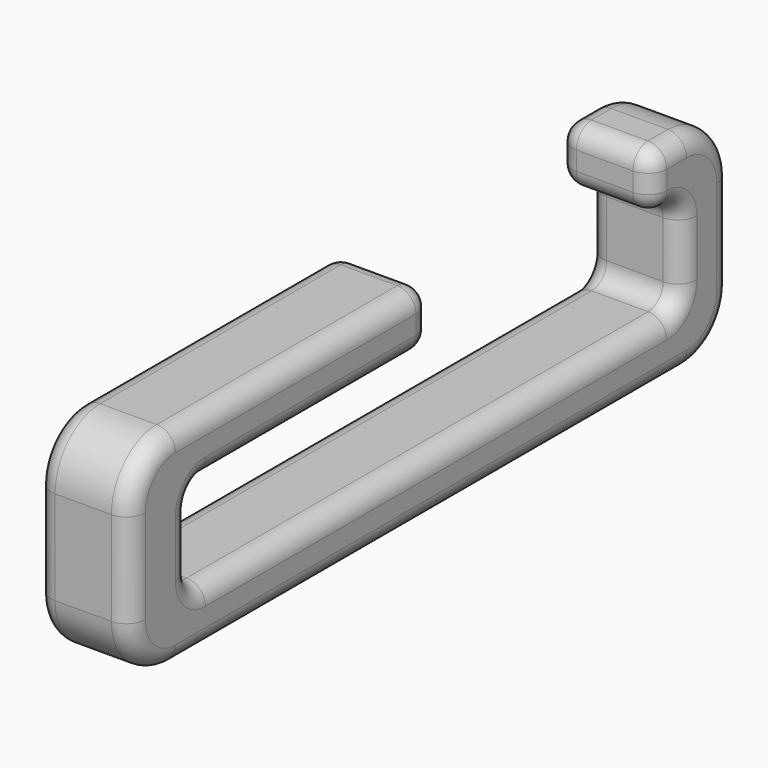
from build123d import *

# Parameters (mm, degrees)
F0_W     = 5
F0_H     = 3.3166247904
F0_H_2   = 16
F0_H_3   = 14.6833752096
F0_H_4   = 2
F1_DEPTH = 3
F2_DEPTH = 11
F3_START = 3
F3_DEPTH = 5
F4_R     = 3
F5_F1_R  = 1
F5_F2_R  = 0.9999


# Not quite as in the source:
# - a fillet or chamfer is up to 0.001 mm smaller than in the source, because OpenCascade refuses the exact size


with BuildPart() as f1:
    # F0 (on Top) → F1 (new body)
    with BuildSketch(Plane.XY):
        Rectangle(F0_W, F0_H)
        with Locations((0, -26.3416876048)):
            Rectangle(F0_W, F0_H_2)
        with Locations((0, -11)):
            Rectangle(F0_W, F0_H_3)
        with Locations((0, -2.6583123952)):
            Rectangle(F0_W, F0_H_4)
        Polygon((2.5, -34.3416876048), (-2.5, -34.3416876048), (-2.5, -38.3416876048), (0, -38.3416876048), (2.5, -38.3416876048), align=None)
    extrude(amount=F1_DEPTH)

    # F0 (on Top) → F2 (join)
    with BuildSketch(Plane.XY):
        Rectangle(F0_W, F0_H)
        with Locations((0, -2.6583123952)):
            Rectangle(F0_W, F0_H_4)
        Polygon((2.5, -34.3416876048), (-2.5, -34.3416876048), (-2.5, -38.3416876048), (0, -38.3416876048), (2.5, -38.3416876048), align=None)
        with Locations((0, -26.3416876048)):
            Rectangle(F0_W, F0_H_2)
    extrude(amount=F2_DEPTH)

    # F0 (on Top) → F3 (cut)
    with BuildSketch(Plane.XY.offset(F3_START)):
        with Locations((0, -2.6583123952)):
            Rectangle(F0_W, F0_H_4)
        with Locations((0, -26.3416876048)):
            Rectangle(F0_W, F0_H_2)
    extrude(amount=F3_DEPTH, mode=Mode.SUBTRACT)

    # F4
    f4_edges = [f1.edges().sort_by_distance(p)[0] for p in [
        (0, 1.658312, 11),
        (0, -38.341688, 11),
        (0, -38.341688, 0),
        (0, 1.658312, 0),
    ]]
    fillet(f4_edges, radius=F4_R)

    # F5: fillet of radius 1 on 16 edges, made by hand

    # F5_f1
    f5_f1_edges = [f1.edges().sort_by_distance(p)[0] for p in [
        (0, -34.3416876048, 8),
        (0, -34.3416876048, 3),
        (0, -1.6583123952, 3),
        (0, -1.6583123952, 8),
    ]]
    fillet(f5_f1_edges, radius=F5_F1_R)

    # F5_f2 (radius 1 in the source; OpenCascade refuses exactly that, so slightly less here)
    f5_f2_edges = [f1.edges().sort_by_distance(p)[0] for p in [
        (-2.5, -26.8416876048, 11),
        (2.5, -26.8416876048, 11),
        (2.5, -3.6583123952, 9.5),
        (0, -3.6583123952, 11),
        (-2.5, -3.6583123952, 9.5),
        (0, -3.6583123952, 8),
        (-2.5, -18.3416876048, 9.5),
        (0, -18.3416876048, 11),
        (2.5, -18.3416876048, 9.5),
        (0, -18.3416876048, 8),
        (2.5, -18, 3),
        (-2.5, -18, 3),
        (2.5, -37.4630079484, 10.1213203436),
        (2.5, -38.3416876048, 5.5),
        (2.5, -37.4630079484, 0.8786796564),
        (2.5, -18.3416876048, 0),
        (2.5, 0.7796327387, 0.8786796564),
        (2.5, 1.6583123952, 5.5),
        (2.5, 0.7796327387, 10.1213203436),
        (2.5, -2.5, 11),
        (-2.5, -37.4630079484, 10.1213203436),
        (-2.5, -38.3416876048, 5.5),
        (-2.5, -37.4630079484, 0.8786796564),
        (-2.5, -18.3416876048, 0),
        (-2.5, 0.7796327387, 0.8786796564),
        (-2.5, 1.6583123952, 5.5),
        (-2.5, 0.7796327387, 10.1213203436),
        (-2.5, -2.5, 11),
        (-2.5, -34.048794386, 3.2928932188),
        (-2.5, -1.951205614, 3.2928932188),
        (2.5, -1.951205614, 3.2928932188),
        (2.5, -34.048794386, 3.2928932188),
    ]]
    fillet(f5_f2_edges, radius=F5_F2_R)


solid = f1.part
